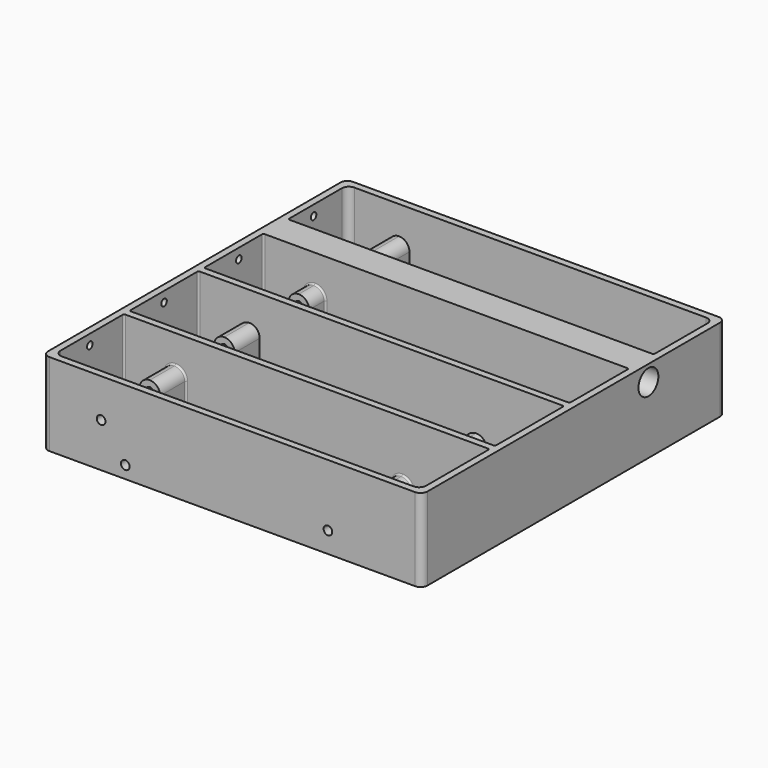
from build123d import *

# Parameters (mm, degrees)
F0_W      = 174.625
F0_H      = 174.625
F1_DEPTH  = 38.1
F2_W      = 168.275
F2_H      = 168.275
F3_DEPTH  = 34.925
F4_R      = 3.175
F5_W      = 167.9709115997
F5_H      = 3.175
F5_W_2    = 168.275
F6_DEPTH  = 38.1
F8_DEPTH  = 5.08
F10_W     = 9.525
F10_H     = 14.859
F11_DEPTH = 25.0952
F12_R     = 4.76249
F13_W     = 9.525
F13_H     = 15.5448
F14_DEPTH = 14.2875
F15_R     = 4.76249
F17_W     = 171.2976
F17_H     = 14.2875
F18_DEPTH = 38.1
F19_R     = 0.762
F20_R     = 5.715
F21_DEPTH = 177.8
F22_W     = 5.08
F22_H     = 5.08
F23_DEPTH = 8.89
F16_R     = 2.0193
F24_DEPTH = 8.89
F9_R      = 1.9939
F25_DEPTH = 177.8
F26_R     = 1.5875
F27_DEPTH = 5.08
F28_R     = 2.0193
F29_DEPTH = 8.2804


# Not quite as in the source:
# - a fillet or chamfer is up to 0.001 mm smaller than in the source, because OpenCascade refuses the exact size


with BuildPart() as f1:
    # F0 (on Top) → F1 (new body)
    with BuildSketch(Plane.XY):
        with Locations((87.3125, 87.3125)):
            Rectangle(F0_W, F0_H)
    extrude(amount=F1_DEPTH)

    # F2 (on face) → F3 (cut)
    with BuildSketch(Plane.XY.offset(38.1)):
        with Locations((87.3125, 87.3125)):
            Rectangle(F2_W, F2_H)
    extrude(amount=-F3_DEPTH, mode=Mode.SUBTRACT)

    # F4
    f4_edges = [f1.edges().sort_by_distance(p)[0] for p in [
        (171.45, 171.45, 20.6375),
        (171.45, 3.175, 20.6375),
        (3.175, 171.45, 20.6375),
        (3.175, 3.175, 20.6375),
        (174.625, 174.625, 19.05),
        (0, 174.625, 19.05),
        (174.625, 0, 19.05),
        (0, 0, 19.05),
    ]]
    fillet(f4_edges, radius=F4_R)

    # F5 (on Top) → F6 (join)
    with BuildSketch(Plane.XY):
        with Locations((87.3412261717, 130.175)):
            Rectangle(F5_W, F5_H)
        with Locations((87.3125, 87.3125)):
            Rectangle(F5_W_2, F5_H)
        with Locations((87.3125, 44.45)):
            Rectangle(F5_W_2, F5_H)
    extrude(amount=F6_DEPTH)

    # F7 (on Top) → F8 (cut)
    with BuildSketch(Plane.XY):
        with BuildLine():
            Line((155.575, 155.0289), (73.025, 155.0289))
            ThreePointArc((73.025, 155.0289), (69.596, 151.5999), (73.025, 148.1709))
            Line((73.025, 148.1709), (155.575, 148.1709))
            ThreePointArc((155.575, 148.1709), (159.004, 151.5999), (155.575, 155.0289))
        make_face()
        with BuildLine():
            Line((73.025, 105.3211), (155.575, 105.3211))
            ThreePointArc((155.575, 105.3211), (159.004, 108.7501), (155.575, 112.1791))
            Line((155.575, 112.1791), (73.025, 112.1791))
            ThreePointArc((73.025, 112.1791), (69.596, 108.7501), (73.025, 105.3211))
        make_face()
        with BuildLine():
            Line((73.025, 62.4713), (155.575, 62.4713))
            ThreePointArc((155.575, 62.4713), (159.004, 65.9003), (155.575, 69.3293))
            Line((155.575, 69.3293), (73.025, 69.3293))
            ThreePointArc((73.025, 69.3293), (69.596, 65.9003), (73.025, 62.4713))
        make_face()
        with BuildLine():
            Line((73.025, 19.6215), (155.575, 19.6215))
            ThreePointArc((155.575, 19.6215), (159.004, 23.0505), (155.575, 26.4795))
            Line((155.575, 26.4795), (73.025, 26.4795))
            ThreePointArc((73.025, 26.4795), (69.596, 23.0505), (73.025, 19.6215))
        make_face()
    extrude(amount=F8_DEPTH, mode=Mode.SUBTRACT)

    # F10 (on Top) → F11 (join)
    with BuildSketch(Plane.XY):
        with Locations((26.9875, 10.6045)):
            Rectangle(F10_W, F10_H)
        with Locations((26.9875, 35.433)):
            Rectangle(F10_W, F10_H)
        with Locations((26.9875, 53.4543)):
            Rectangle(F10_W, F10_H)
        with Locations((26.9875, 78.2828)):
            Rectangle(F10_W, F10_H)
        with Locations((26.9875, 96.3041)):
            Rectangle(F10_W, F10_H)
        with Locations((26.9875, 121.1326)):
            Rectangle(F10_W, F10_H)
        with Locations((26.9875, 139.1539)):
            Rectangle(F10_W, F10_H)
        with Locations((26.9875, 163.9824)):
            Rectangle(F10_W, F10_H)
    extrude(amount=F11_DEPTH)

    # F12 (radius 4.7625 in the source; OpenCascade refuses exactly that, so slightly less here)
    f12_edges = [f1.edges().sort_by_distance(p)[0] for p in [
        (22.225, 163.9824, 25.0952),
        (31.75, 163.9824, 25.0952),
        (31.75, 139.17295, 25.0952),
        (22.225, 139.17295, 25.0952),
        (31.75, 121.1326, 25.0952),
        (31.75, 96.3168, 25.0952),
        (31.75, 78.2828, 25.0952),
        (31.75, 53.46065, 25.0952),
        (31.75, 35.433, 25.0952),
        (31.75, 10.6045, 25.0952),
        (22.225, 121.1326, 25.0952),
        (22.225, 78.2828, 25.0952),
        (22.225, 96.3168, 25.0952),
        (22.225, 53.46065, 25.0952),
        (22.225, 35.433, 25.0952),
        (22.225, 10.6045, 25.0952),
    ]]
    fillet(f12_edges, radius=F12_R)

    # F13 (on face) → F14 (join)
    with BuildSketch(Plane(origin=(0, 0, 0), x_dir=(1, 0, 0), z_dir=(0, 0, -1))):
        with Locations((131.3561, -10.9474)):
            Rectangle(F13_W, F13_H)
        with Locations((131.3561, -35.0901)):
            Rectangle(F13_W, F13_H)
        with Locations((131.3561, -53.7972)):
            Rectangle(F13_W, F13_H)
        with Locations((131.3561, -77.9399)):
            Rectangle(F13_W, F13_H)
        with Locations((131.3561, -96.647)):
            Rectangle(F13_W, F13_H)
        with Locations((131.3561, -120.7897)):
            Rectangle(F13_W, F13_H)
        with Locations((131.3561, -139.4968)):
            Rectangle(F13_W, F13_H)
        with Locations((131.3561, -163.6395)):
            Rectangle(F13_W, F13_H)
    extrude(amount=-F14_DEPTH)

    # F15 (radius 4.7625 in the source; OpenCascade refuses exactly that, so slightly less here)
    f15_edges = [f1.edges().sort_by_distance(p)[0] for p in [
        (126.5936, 163.6395, 14.2875),
        (126.5936, 139.51585, 14.2875),
        (126.5936, 120.7897, 14.2875),
        (126.5936, 96.6597, 14.2875),
        (126.5936, 77.9399, 14.2875),
        (126.5936, 53.80355, 14.2875),
        (126.5936, 35.0901, 14.2875),
        (126.5936, 10.9474, 14.2875),
        (136.1186, 10.9474, 14.2875),
        (136.1186, 35.0901, 14.2875),
        (136.1186, 53.80355, 14.2875),
        (136.1186, 77.9399, 14.2875),
        (136.1186, 96.6597, 14.2875),
        (136.1186, 120.7897, 14.2875),
        (136.1186, 139.51585, 14.2875),
        (136.1186, 163.6395, 14.2875),
    ]]
    fillet(f15_edges, radius=F15_R)

    # F17 (on Top) → F18 (join)
    with BuildSketch(Plane.XY):
        with Locations((88.2789392626, 130.16865)):
            Rectangle(F17_W, F17_H)
    extrude(amount=F18_DEPTH)

    # F19
    f19_edges = [f1.edges().sort_by_distance(p)[0] for p in [
        (31.75, 137.3124, 11.753855),
        (126.5936, 137.3124, 6.350005),
        (31.75, 123.0249, 11.753855),
        (136.1186, 123.0249, 6.350005),
        (136.1186, 85.7123, 6.350005),
        (31.75, 85.7123, 11.753855),
        (31.75, 42.8625, 11.753855),
        (136.1186, 42.8625, 6.350005),
        (3.175, 42.8625, 20.6375),
        (3.175, 85.725, 20.6375),
        (3.175, 123.0249, 20.6375),
        (171.45, 168.275, 20.6375),
        (171.45, 123.0249, 20.6375),
        (171.45, 85.725, 20.6375),
        (171.45, 42.8625, 20.6375),
        (136.1186, 88.9, 6.350005),
        (31.75, 88.9, 11.753855),
        (31.75, 46.0375, 11.753855),
        (136.1186, 46.0375, 6.350005),
        (136.1186, 3.175, 6.350005),
        (31.75, 3.175, 11.753855),
        (3.175, 46.0375, 20.6375),
        (3.175, 88.9, 20.6375),
        (171.45, 46.0375, 20.6375),
        (171.45, 88.9, 20.6375),
        (171.45, 137.3124, 20.6375),
        (3.175, 168.275, 20.6375),
        (3.175, 137.3124, 20.6375),
        (134.723699, 3.175, 12.892599),
        (131.3561, 3.175, 14.2875),
        (127.988501, 3.175, 12.892599),
        (126.5936, 3.175, 6.350005),
        (22.225, 3.175, 11.753855),
        (30.355099, 3.175, 23.700299),
        (23.619901, 3.175, 23.700299),
        (26.9875, 3.175, 25.0952),
        (126.5936, 42.8625, 6.350005),
        (127.988501, 42.8625, 12.892599),
        (131.3561, 42.8625, 14.2875),
        (134.723699, 42.8625, 12.892599),
        (30.355099, 42.8625, 23.700299),
        (26.9875, 42.8625, 25.0952),
        (23.619901, 42.8625, 23.700299),
        (22.225, 42.8625, 11.753855),
        (134.723699, 46.0375, 12.892599),
        (131.3561, 46.0375, 14.2875),
        (127.988501, 46.0375, 12.892599),
        (126.5936, 46.0375, 6.350005),
        (22.225, 46.0375, 11.753855),
        (30.355099, 46.0375, 23.700299),
        (23.619901, 46.0375, 23.700299),
        (26.9875, 46.0375, 25.0952),
        (134.723699, 88.9, 12.892599),
        (131.3561, 88.9, 14.2875),
        (127.988501, 88.9, 12.892599),
        (126.5936, 88.9, 6.350005),
        (22.225, 88.9, 11.753855),
        (30.355099, 88.9, 23.700299),
        (23.619901, 88.9, 23.700299),
        (26.9875, 88.9, 25.0952),
        (22.225, 123.0249, 11.753855),
        (23.619901, 123.0249, 23.700299),
        (26.9875, 123.0249, 25.0952),
        (30.355099, 123.0249, 23.700299),
        (126.5936, 123.0249, 6.350005),
        (127.988501, 123.0249, 12.892599),
        (131.3561, 123.0249, 14.2875),
        (134.723699, 123.0249, 12.892599),
        (136.1186, 137.3124, 6.350005),
        (134.723699, 137.3124, 12.892599),
        (131.3561, 137.3124, 14.2875),
        (127.988501, 137.3124, 12.892599),
        (30.355099, 137.3124, 23.700299),
        (26.9875, 137.3124, 25.0952),
        (23.619901, 137.3124, 23.700299),
        (22.225, 137.3124, 11.753855),
        (22.225, 85.7123, 11.753855),
        (23.619901, 85.7123, 23.700299),
        (26.9875, 85.7123, 25.0952),
        (30.355099, 85.7123, 23.700299),
        (134.723699, 85.7123, 12.892599),
        (131.3561, 85.7123, 14.2875),
        (126.5936, 85.7123, 6.350005),
        (127.988501, 85.7123, 12.892599),
    ]]
    fillet(f19_edges, radius=F19_R)

    # F20 (on face) → F21 (cut)
    with BuildSketch(Plane(origin=(0, 0, 0), x_dir=(0, -1, 0), z_dir=(-1, 0, 0))):
        with Locations((-130.2791535854, 30.7504776865)):
            Circle(F20_R)
    extrude(amount=-F21_DEPTH, mode=Mode.SUBTRACT)

    # F22 (on face) → F23 (join)
    with BuildSketch(Plane(origin=(0, 0, 0), x_dir=(1, 0, 0), z_dir=(0, 0, -1))):
        with Locations((38.1, -5.715)):
            Rectangle(F22_W, F22_H)
        with Locations((38.1, -168.91)):
            Rectangle(F22_W, F22_H)
    extrude(amount=-F23_DEPTH)

    # F16 (on face) → F24 (cut)
    with BuildSketch(Plane.XZ):
        with Locations((38.1, 5.715)):
            Circle(F16_R)
    extrude(amount=-F24_DEPTH, mode=Mode.SUBTRACT)

    # F9 (on face) → F25 (cut)
    with BuildSketch(Plane.XZ):
        with Locations((131.3561, 9.525)):
            Circle(F9_R)
        with Locations((26.9875, 20.32)):
            Circle(F9_R)
    extrude(amount=-F25_DEPTH, mode=Mode.SUBTRACT)

    # F26 (on face) → F27 (cut)
    with BuildSketch(Plane(origin=(0, 0, 0), x_dir=(0, -1, 0), z_dir=(-1, 0, 0))):
        with Locations((-151.985630393, 33.3804748952)):
            Circle(F26_R)
        with Locations((-108.972735703, 33.3804748952)):
            Circle(F26_R)
        with Locations((-65.959841013, 33.3804748952)):
            Circle(F26_R)
        with Locations((-23.2477318496, 33.3804748952)):
            Circle(F26_R)
    extrude(amount=-F27_DEPTH, mode=Mode.SUBTRACT)

    # F28 (on face) → F29 (cut)
    with BuildSketch(Plane(origin=(0, 174.625, 0), x_dir=(-1, 0, 0), z_dir=(0, 1, 0))):
        with Locations((-38.098141551, 5.7257381268)):
            Circle(F28_R)
    extrude(amount=-F29_DEPTH, mode=Mode.SUBTRACT)


solid = f1.part
